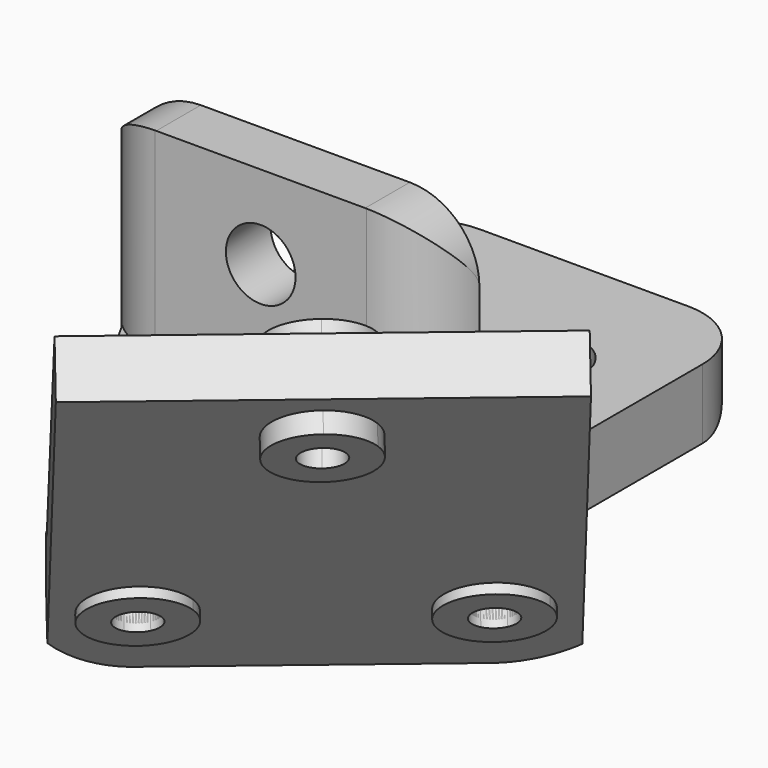
from build123d import *

# Parameters (mm, degrees)
F0_W           = 25
F0_H           = 25
F0_R           = 3
F1_DEPTH       = 5
F0_H_2         = 4
F2_DEPTH       = 18
F3_DEPTH       = 5
F4_R           = 2.5
F5_DEPTH       = 4
F7_DEPTH       = 4
F8_W           = 30
F8_H           = 8
F9_DEPTH       = 1
F11_DEPTH      = 30
F12_T1_DEPTH   = 50
F12_T3_DEPTH   = 30
F12_2_T1_DEPTH = 42.4948974279
F12_2_T3_DEPTH = 29
F12_3_T1_DEPTH = 29.4948974279
F12_4_F1_R     = 5
F12_4_F2_R     = 5
F14_DEPTH      = 1.5
F15_DEPTH      = 10
F14_FACE_R     = 3.5
F14_FACE_R_2   = 1.5
F16_DEPTH      = 10
F17_DEPTH      = 5.5


# Not quite as in the source:
# - a fillet or chamfer that OpenCascade refuses, or shapes differently, is made with other operations: its cross-section is extruded or revolved along the edge and cut away or added


with BuildPart() as f1:
    # F0 (on Top) → F1 (new body)
    with BuildSketch(Plane.XY):
        with Locations((0, 12.5)):
            Rectangle(F0_W, F0_H)
        with Locations((5, 15)):
            Circle(F0_R, mode=Mode.SUBTRACT)
    extrude(amount=-F1_DEPTH)

    # F12: fillet of radius 5 on 3 edges, made by hand

    # F12_s2 → F12_t1 (cut)
    with BuildSketch(Plane.YZ.offset(-25)):
        with BuildLine():
            ThreePointArc((25, 0), (23.5355339059, -3.5355339059), (20, -5))
            Line((20, -5), (25, -5))
            Line((25, -5), (25, 0))
        make_face()
    extrude(amount=F12_T1_DEPTH, mode=Mode.SUBTRACT)

    # F12_s4 → F12_t3 (cut)
    with BuildSketch(Plane.XY.offset(-17.5)):
        with BuildLine():
            ThreePointArc((12.5, 20), (11.0355339059, 23.5355339059), (7.5, 25))
            Line((7.5, 25), (12.5, 25))
            Line((12.5, 25), (12.5, 20))
        make_face()
        with BuildLine():
            ThreePointArc((-12.5, 20), (-11.0355339059, 23.5355339059), (-7.5, 25))
            Line((-7.5, 25), (-12.5, 25))
            Line((-12.5, 25), (-12.5, 20))
        make_face()
    extrude(amount=F12_T3_DEPTH, mode=Mode.SUBTRACT)


with BuildPart() as f2:
    # F0 (on Top) → F2 (new body)
    with BuildSketch(Plane.XY):
        with Locations((0, -2)):
            Rectangle(F0_W, F0_H_2)
    extrude(amount=F2_DEPTH)


with BuildPart() as f3:
    # F3 (new): a face of the model
    f3_faces = [f2.part.faces().sort_by_distance(p)[0] for p in [
        (0, -2, 0),
    ]]
    extrude(f3_faces, amount=F3_DEPTH)

    # F12#3: fillet of radius 5 on 1 edges, made by hand

    # F12_3_s2 → F12_3_t1 (cut)
    with BuildSketch(Plane.XY.offset(-17.2474487139)):
        with BuildLine():
            ThreePointArc((7.6010205144, -4), (10.7632981746, -2.8729833462), (12.5, 0))
            Line((12.5, 0), (12.5, -4))
            Line((12.5, -4), (7.6010205144, -4))
        make_face()
    extrude(amount=F12_3_T1_DEPTH, mode=Mode.SUBTRACT)


with BuildPart() as f2_1:
    add(f2.part)

    # F4 (on face) → F5 (cut)
    with BuildSketch(Plane(origin=(0, 0, 0), x_dir=(-1, 0, 0), z_dir=(0, 1, 0))):
        with Locations((0, 12)):
            Circle(F4_R)
    extrude(amount=-F5_DEPTH, mode=Mode.SUBTRACT)

    # F12#2: fillet of radius 5 on 4 edges, made by hand

    # F12_2_s2 → F12_2_t1 (cut)
    with BuildSketch(Plane.XY.offset(-12.2474487139)):
        with BuildLine():
            ThreePointArc((12.5, 0), (10.7632981746, -2.8729833462), (7.6010205144, -4))
            Line((7.6010205144, -4), (12.5, -4))
            Line((12.5, -4), (12.5, 0))
        make_face()
        with BuildLine():
            ThreePointArc((-12.5, 0), (-10.7632981746, -2.8729833462), (-7.6010205144, -4))
            Line((-7.6010205144, -4), (-12.5, -4))
            Line((-12.5, -4), (-12.5, 0))
        make_face()
    extrude(amount=F12_2_T1_DEPTH, mode=Mode.SUBTRACT)

    # F12_2_s4 → F12_2_t3 (cut)
    with BuildSketch(Plane.XZ.offset(-12.5)):
        with BuildLine():
            ThreePointArc((-7.5, 18), (-11.0355339059, 16.5355339059), (-12.5, 13))
            Line((-12.5, 13), (-12.5, 18))
            Line((-12.5, 18), (-7.5, 18))
        make_face()
        with BuildLine():
            ThreePointArc((12.5, 13), (11.0355339059, 16.5355339059), (7.5, 18))
            Line((7.5, 18), (12.5, 18))
            Line((12.5, 18), (12.5, 13))
        make_face()
    extrude(amount=F12_2_T3_DEPTH, mode=Mode.SUBTRACT)


with BuildPart() as f7:
    # F6 (on Top) → F7 (new body, symmetric)
    with BuildSketch(Plane.XY):
        Polygon((12.8557521937, -15.3208888624), (0, 0), (-12.5, 0), (1.3650855469, -24.9627030077), align=None)
        Polygon((12.5, 0), (0, 0), (12.8557521937, -15.3208888624), (24.3464188405, -5.6790747171), align=None)
    extrude(amount=F7_DEPTH, both=True)

    # F8 (on face) → F9 (join)
    with BuildSketch(Plane(origin=(12.8557521937, -15.3208888624, 0), x_dir=(0.7660444431, 0.6427876097, 0), z_dir=(0.6427876097, -0.7660444431, 0))):
        Rectangle(F8_W, F8_H)
    extrude(amount=F9_DEPTH)

    # F10 (on face) → F11 (join, through all)
    with BuildSketch(Plane(origin=(11.4906666468, 9.6418141453, 0), x_dir=(-0.6427876097, 0.7660444431, 0), z_dir=(0.7660444431, 0.6427876097, 0))):
        Polygon((-21, -4), (-21, 4), (-40.2836282906, 26.9813332936), (-43.3478060631, 24.4101828548), align=None)
    extrude(amount=-F11_DEPTH)

    # F12#4: fillet of radius 5 on 2 edges, made by hand

    # F12_4_f1
    f12_4_f1_edges = [f7.edges().sort_by_distance(p)[0] for p in [
        (-5.5674572265, -12.4813515038, -4),
    ]]
    fillet(f12_4_f1_edges, radius=F12_4_F1_R)

    # F12_4_f2
    f12_4_f2_edges = [f7.edges().sort_by_distance(p)[0] for p in [
        (18.4232094203, -2.8395373585, -4),
    ]]
    fillet(f12_4_f2_edges, radius=F12_4_F2_R)

    # F13 (on face) → F15 (cut, symmetric)
    with BuildSketch(Plane(origin=(6.6552238776, -7.9313869657, -8.687777762), x_dir=(0.8703668321, 0.3319915759, 0.3636525418), z_dir=(-0.4924038765, 0.5868240888, 0.6427876097))):
        with BuildLine():
            ThreePointArc((19.0183601074, -35.2607900987), (18.4102225056, -37.293071737), (20.4425041439, -37.9012093388))
            Line((20.4425041439, -37.9012093388), (19.7304321257, -36.5809997188))
            Line((19.7304321257, -36.5809997187), (19.0183601074, -35.2607900987))
        make_face()
        with BuildLine():
            Line((19.7304321257, -36.5809997188), (20.4425041439, -37.9012093388))
            ThreePointArc((20.4425041439, -37.9012093388), (21.0184748321, -37.3497298315), (21.2304321257, -36.5809997188))
            ThreePointArc((21.2304321257, -36.5809997188), (20.4991622385, -35.2929570123), (19.0183601074, -35.2607900987))
            Line((19.0183601074, -35.2607900987), (19.7304321257, -36.5809997187))
        make_face()
        with BuildLine():
            Line((-0.280196035, -18.969408903), (-1.5974685891, -19.679896777))
            ThreePointArc((-1.5974685891, -19.679896777), (-0.7317958781, -21.9116872473), (1.1782967704, -20.4688345106))
            ThreePointArc((1.1782967704, -20.4688345106), (0.7535318126, -19.4229522974), (-0.280196035, -18.969408903))
        make_face()
        with BuildLine():
            ThreePointArc((-0.280196035, -18.969408903), (-1.0337752479, -19.1486248906), (-1.5974685891, -19.679896777))
            Line((-1.5974685891, -19.679896777), (-0.280196035, -18.969408903))
        make_face()
        with BuildLine():
            Line((16.0053263446, -10.1856032003), (17.3225988986, -9.4751153263))
            ThreePointArc((17.3225988986, -9.4751153263), (16.5690196858, -9.6543313139), (16.0053263446, -10.1856032003))
        make_face()
        with BuildLine():
            ThreePointArc((18.7810917041, -10.9745409339), (18.3563267462, -9.9286587206), (17.3225988986, -9.4751153263))
            Line((17.3225988986, -9.4751153263), (16.0053263446, -10.1856032003))
            ThreePointArc((16.0053263446, -10.1856032003), (15.7817488172, -10.9301460285), (15.960882084, -11.6866129522))
            ThreePointArc((15.960882084, -11.6866129522), (17.6483011606, -12.4288989418), (18.7810917041, -10.9745409339))
        make_face()
    extrude(amount=F15_DEPTH, both=True, mode=Mode.SUBTRACT)

    # F14_face (on face) → F16 (cut)
    with BuildSketch(Plane(origin=(5.636618242, -22.2746983085, 5.9600391905), x_dir=(0.8703668321, 0.3319915759, 0.3636525418), z_dir=(-0.4924038765, 0.5868240888, 0.6427876097))):
        Circle(F14_FACE_R)
        Circle(F14_FACE_R_2, mode=Mode.SUBTRACT)
        with Locations((20.0521353553, -16.1121652081)):
            Circle(F14_FACE_R)
        with Locations((20.0521353553, -16.1121652081)):
            Circle(F14_FACE_R_2, mode=Mode.SUBTRACT)
        with Locations((17.6027949337, 9.4942935767)):
            Circle(F14_FACE_R)
        with Locations((17.6027949337, 9.4942935767)):
            Circle(F14_FACE_R_2, mode=Mode.SUBTRACT)
    extrude(amount=F16_DEPTH, mode=Mode.SUBTRACT)


with BuildPart() as f14:
    # F13 (on face) → F14 (new body)
    with BuildSketch(Plane(origin=(6.6552238776, -7.9313869657, -8.687777762), x_dir=(0.8703668321, 0.3319915759, 0.3636525418), z_dir=(-0.4924038765, 0.5868240888, 0.6427876097))):
        with BuildLine():
            ThreePointArc((18.0689307498, -33.5005106053), (16.6499430123, -38.2425010947), (21.3919335016, -39.6614888321))
            Line((21.3919335016, -39.6614888321), (20.4425041439, -37.9012093388))
            ThreePointArc((20.4425041439, -37.9012093388), (18.4102225056, -37.293071737), (19.0183601074, -35.2607900987))
            Line((19.0183601074, -35.2607900987), (18.0689307498, -33.5005106053))
        make_face()
        with BuildLine():
            Line((20.4425041439, -37.9012093388), (21.3919335016, -39.6614888321))
            ThreePointArc((21.3919335016, -39.6614888321), (22.7358651074, -38.3747033153), (23.2304321257, -36.5809997188))
            ThreePointArc((23.2304321257, -36.5809997188), (21.5241357222, -33.575566737), (18.0689307498, -33.5005106053))
            Line((18.0689307498, -33.5005106053), (19.0183601074, -35.2607900987))
            ThreePointArc((19.0183601074, -35.2607900987), (20.4991622385, -35.2929570123), (21.2304321257, -36.5809997188))
            ThreePointArc((21.2304321257, -36.5809997188), (21.0184748321, -37.3497298315), (20.4425041439, -37.9012093388))
        make_face()
    extrude(amount=F14_DEPTH)


with BuildPart() as f14b:
    # F13 (on face) → F14, piece 2 (new body)
    with BuildSketch(Plane(origin=(6.6552238776, -7.9313869657, -8.687777762), x_dir=(0.8703668321, 0.3319915759, 0.3636525418), z_dir=(-0.4924038765, 0.5868240888, 0.6427876097))):
        with BuildLine():
            ThreePointArc((20.7810917041, -10.9745409339), (20.4513009209, -9.4913775842), (19.524078263, -8.2877191504))
            Line((19.524078263, -8.2877191504), (17.3225988986, -9.4751153263))
            ThreePointArc((17.3225988986, -9.4751153263), (18.3563267462, -9.9286587206), (18.7810917041, -10.9745409339))
            ThreePointArc((18.7810917041, -10.9745409339), (17.6483011606, -12.4288989418), (15.960882084, -11.6866129522))
            Line((15.960882084, -11.6866129522), (14.2006025907, -12.6360423098))
            ThreePointArc((14.2006025907, -12.6360423098), (18.1379137693, -14.3680429522), (20.7810917041, -10.9745409339))
        make_face()
        with BuildLine():
            Line((17.3225988986, -9.4751153263), (19.524078263, -8.2877191504))
            ThreePointArc((19.524078263, -8.2877191504), (15.6195903281, -7.8940518205), (13.8038469802, -11.3729993761))
            Line((13.8038469802, -11.3729993761), (16.0053263446, -10.1856032003))
            ThreePointArc((16.0053263446, -10.1856032003), (16.5690196858, -9.6543313139), (17.3225988986, -9.4751153263))
        make_face()
        with BuildLine():
            ThreePointArc((13.8038469802, -11.3729993761), (13.9419619322, -12.0234510191), (14.2006025907, -12.6360423098))
            Line((14.2006025907, -12.6360423098), (15.960882084, -11.6866129522))
            ThreePointArc((15.960882084, -11.6866129522), (15.7817488172, -10.9301460285), (16.0053263446, -10.1856032003))
            Line((16.0053263446, -10.1856032003), (13.8038469802, -11.3729993761))
        make_face()
    extrude(amount=F14_DEPTH)


with BuildPart() as f14c:
    # F13 (on face) → F14, piece 3 (new body)
    with BuildSketch(Plane(origin=(6.6552238776, -7.9313869657, -8.687777762), x_dir=(0.8703668321, 0.3319915759, 0.3636525418), z_dir=(-0.4924038765, 0.5868240888, 0.6427876097))):
        with BuildLine():
            Line((-1.5974685891, -19.679896777), (-3.7989479535, -20.8672929529))
            ThreePointArc((-3.7989479535, -20.8672929529), (-0.1221493943, -23.9631410608), (3.1782967704, -20.4688345106))
            ThreePointArc((3.1782967704, -20.4688345106), (2.8485059872, -18.985671161), (1.9212833294, -17.7820127271))
            Line((1.9212833294, -17.7820127271), (-0.280196035, -18.969408903))
            ThreePointArc((-0.280196035, -18.969408903), (0.7535318126, -19.4229522974), (1.1782967704, -20.4688345106))
            ThreePointArc((1.1782967704, -20.4688345106), (-0.7317958781, -21.9116872473), (-1.5974685891, -19.679896777))
        make_face()
        with BuildLine():
            ThreePointArc((1.9212833294, -17.7820127271), (-1.9832046056, -17.3883453972), (-3.7989479535, -20.8672929529))
            Line((-3.7989479535, -20.8672929529), (-1.5974685891, -19.679896777))
            ThreePointArc((-1.5974685891, -19.679896777), (-1.0337752479, -19.1486248906), (-0.280196035, -18.969408903))
            Line((-0.280196035, -18.969408903), (1.9212833294, -17.7820127271))
        make_face()
    extrude(amount=F14_DEPTH)


with BuildPart() as f17:
    # F13 (on face) → F17 (new body)
    with BuildSketch(Plane(origin=(6.6552238776, -7.9313869657, -8.687777762), x_dir=(0.8703668321, 0.3319915759, 0.3636525418), z_dir=(-0.4924038765, 0.5868240888, 0.6427876097))):
        with BuildLine():
            ThreePointArc((18.0689307498, -33.5005106053), (16.6499430123, -38.2425010947), (21.3919335016, -39.6614888321))
            Line((21.3919335016, -39.6614888321), (20.4425041439, -37.9012093388))
            ThreePointArc((20.4425041439, -37.9012093388), (18.4102225056, -37.293071737), (19.0183601074, -35.2607900987))
            Line((19.0183601074, -35.2607900987), (18.0689307498, -33.5005106053))
        make_face()
        with BuildLine():
            Line((20.4425041439, -37.9012093388), (21.3919335016, -39.6614888321))
            ThreePointArc((21.3919335016, -39.6614888321), (22.7358651074, -38.3747033153), (23.2304321257, -36.5809997188))
            ThreePointArc((23.2304321257, -36.5809997188), (21.5241357222, -33.575566737), (18.0689307498, -33.5005106053))
            Line((18.0689307498, -33.5005106053), (19.0183601074, -35.2607900987))
            ThreePointArc((19.0183601074, -35.2607900987), (20.4991622385, -35.2929570123), (21.2304321257, -36.5809997188))
            ThreePointArc((21.2304321257, -36.5809997188), (21.0184748321, -37.3497298315), (20.4425041439, -37.9012093388))
        make_face()
    extrude(amount=-F17_DEPTH)


with BuildPart() as f17b:
    # F13 (on face) → F17, piece 2 (new body)
    with BuildSketch(Plane(origin=(6.6552238776, -7.9313869657, -8.687777762), x_dir=(0.8703668321, 0.3319915759, 0.3636525418), z_dir=(-0.4924038765, 0.5868240888, 0.6427876097))):
        with BuildLine():
            Line((-1.5974685891, -19.679896777), (-3.7989479535, -20.8672929529))
            ThreePointArc((-3.7989479535, -20.8672929529), (-0.1221493943, -23.9631410608), (3.1782967704, -20.4688345106))
            ThreePointArc((3.1782967704, -20.4688345106), (2.8485059872, -18.985671161), (1.9212833294, -17.7820127271))
            Line((1.9212833294, -17.7820127271), (-0.280196035, -18.969408903))
            ThreePointArc((-0.280196035, -18.969408903), (0.7535318126, -19.4229522974), (1.1782967704, -20.4688345106))
            ThreePointArc((1.1782967704, -20.4688345106), (-0.7317958781, -21.9116872473), (-1.5974685891, -19.679896777))
        make_face()
        with BuildLine():
            ThreePointArc((1.9212833294, -17.7820127271), (-1.9832046056, -17.3883453972), (-3.7989479535, -20.8672929529))
            Line((-3.7989479535, -20.8672929529), (-1.5974685891, -19.679896777))
            ThreePointArc((-1.5974685891, -19.679896777), (-1.0337752479, -19.1486248906), (-0.280196035, -18.969408903))
            Line((-0.280196035, -18.969408903), (1.9212833294, -17.7820127271))
        make_face()
    extrude(amount=-F17_DEPTH)


with BuildPart() as f17c:
    # F13 (on face) → F17, piece 3 (new body)
    with BuildSketch(Plane(origin=(6.6552238776, -7.9313869657, -8.687777762), x_dir=(0.8703668321, 0.3319915759, 0.3636525418), z_dir=(-0.4924038765, 0.5868240888, 0.6427876097))):
        with BuildLine():
            Line((17.3225988986, -9.4751153263), (19.524078263, -8.2877191504))
            ThreePointArc((19.524078263, -8.2877191504), (15.6195903281, -7.8940518205), (13.8038469802, -11.3729993761))
            Line((13.8038469802, -11.3729993761), (16.0053263446, -10.1856032003))
            ThreePointArc((16.0053263446, -10.1856032003), (16.5690196858, -9.6543313139), (17.3225988986, -9.4751153263))
        make_face()
        with BuildLine():
            ThreePointArc((20.7810917041, -10.9745409339), (20.4513009209, -9.4913775842), (19.524078263, -8.2877191504))
            Line((19.524078263, -8.2877191504), (17.3225988986, -9.4751153263))
            ThreePointArc((17.3225988986, -9.4751153263), (18.3563267462, -9.9286587206), (18.7810917041, -10.9745409339))
            ThreePointArc((18.7810917041, -10.9745409339), (17.6483011606, -12.4288989418), (15.960882084, -11.6866129522))
            Line((15.960882084, -11.6866129522), (14.2006025907, -12.6360423098))
            ThreePointArc((14.2006025907, -12.6360423098), (18.1379137693, -14.3680429522), (20.7810917041, -10.9745409339))
        make_face()
        with BuildLine():
            ThreePointArc((13.8038469802, -11.3729993761), (13.9419619322, -12.0234510191), (14.2006025907, -12.6360423098))
            Line((14.2006025907, -12.6360423098), (15.960882084, -11.6866129522))
            ThreePointArc((15.960882084, -11.6866129522), (15.7817488172, -10.9301460285), (16.0053263446, -10.1856032003))
            Line((16.0053263446, -10.1856032003), (13.8038469802, -11.3729993761))
        make_face()
    extrude(amount=-F17_DEPTH)


solid = Compound([f1.part, f3.part, f2_1.part, f7.part, f14.part, f14b.part, f14c.part, f17.part, f17b.part, f17c.part])
